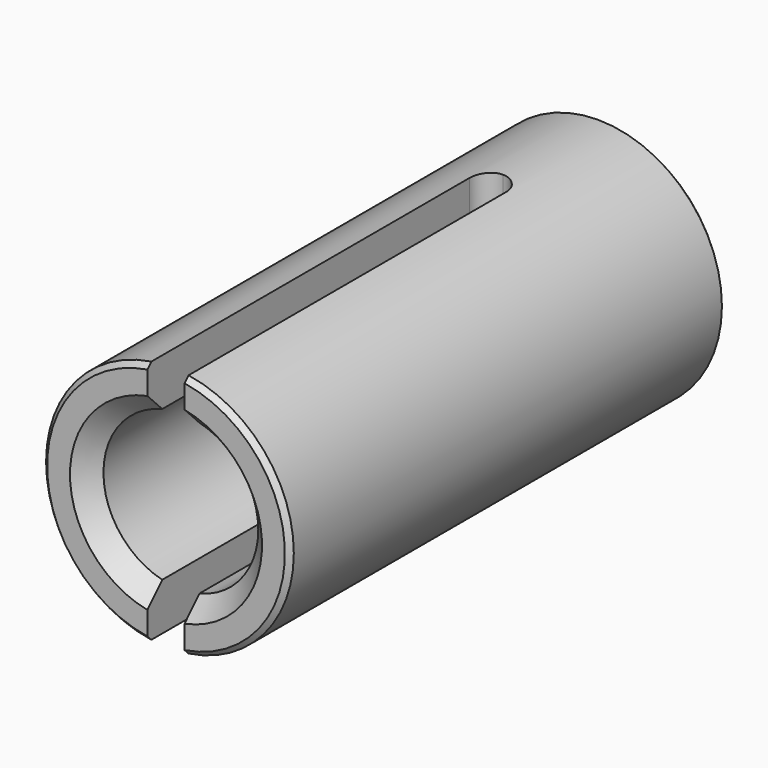
from build123d import *

# Parameters (mm, degrees)
F0_R     = 5
F0_R_2   = 3.125
F1_DEPTH = 22
F3_DEPTH = 17
F4_SIZE  = 0.2
F5_SIZE  = 0.75
F6_R     = 0.7499


# Not quite as in the source:
# - a fillet or chamfer is up to 0.001 mm smaller than in the source, because OpenCascade refuses the exact size


with BuildPart() as f1:
    # F0 (on Front) → F1 (new body)
    with BuildSketch(Plane.XZ):
        Circle(F0_R)
        Circle(F0_R_2, mode=Mode.SUBTRACT)
    extrude(amount=F1_DEPTH)

    # F2 (on face) → F3 (cut)
    with BuildSketch(Plane.XZ.offset(22)):
        with BuildLine():
            ThreePointArc((0.75, 4.9434299833), (0, 5), (-0.75, 4.9434299833))
            Line((-0.75, 4.9434299833), (-0.75, 3.0336652749))
            ThreePointArc((-0.75, 3.0336652749), (0, 3.125), (0.75, 3.0336652749))
            Line((0.75, 3.0336652749), (0.75, 4.9434299833))
        make_face()
        with BuildLine():
            ThreePointArc((-0.75, -4.9434299833), (0, -5), (0.75, -4.9434299833))
            Line((0.75, -4.9434299833), (0.75, -3.0336652749))
            ThreePointArc((0.75, -3.0336652749), (0, -3.125), (-0.75, -3.0336652749))
            Line((-0.75, -3.0336652749), (-0.75, -4.9434299833))
        make_face()
    extrude(amount=-F3_DEPTH, mode=Mode.SUBTRACT)

    # F4
    f4_edges = [f1.edges().sort_by_distance(p)[0] for p in [
        (-5, 0, 0),
        (-5, -22, 0),
        (3.791438, -22, -3.259601),
        (-3.125, 0, 0),
    ]]
    chamfer(f4_edges, length=F4_SIZE)

    # F5
    f5_edges = [f1.edges().sort_by_distance(p)[0] for p in [
        (-3.125, -22, 0),
        (2.460627, -22, -1.926379),
    ]]
    chamfer(f5_edges, length=F5_SIZE)

    # F6 (radius 0.75 in the source; OpenCascade refuses exactly that, so slightly less here)
    f6_edges = [f1.edges().sort_by_distance(p)[0] for p in [
        (0.75, -5, -3.988548),
        (-0.75, -5, 3.988548),
        (-0.75, -5, -3.988548),
        (0.75, -5, 3.988548),
    ]]
    fillet(f6_edges, radius=F6_R)


solid = f1.part
